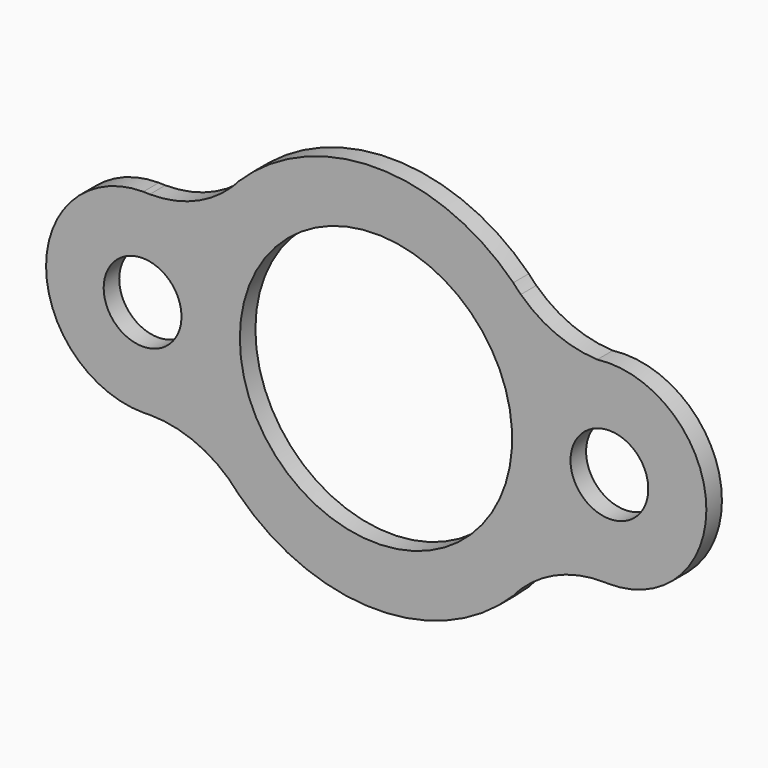
from build123d import *

# Parameters (mm, degrees)
F2_DEPTH = 6.35
F3_D     = 25.4
F4_D     = 88.9


# Not quite as in the source:
# - a length typed as a fraction of an inch, garbled in the dataset ("3 / 203.2 mm" for 3/8 in), is restored


with BuildPart() as f2:
    # F1 (on Front) → F2 (new body)
    with BuildSketch(Plane.XZ):
        with BuildLine():
            ThreePointArc((-47.2755417472, 42.3942574403), (-59.5317634989, 34.5003362533), (-73.8557984397, 31.7890660068))
            ThreePointArc((-73.8557984397, 31.7890660068), (-74.9040664455, 31.8092594153), (-75.9513814682, 31.8582984692))
            ThreePointArc((-75.9513814682, 31.8582984692), (-107.7013814682, 0.1082984692), (-75.9513814682, -31.6417015308))
            ThreePointArc((-75.9513814682, -31.6417015308), (-74.9868907208, -31.6001278987), (-74.0216562697, -31.5830041335))
            ThreePointArc((-74.0216562697, -31.5830041335), (-59.7325831056, -34.2859814401), (-47.4971337693, -42.1458464357))
            ThreePointArc((-47.4971337693, -42.1458464357), (-46.1209982776, -43.530970971), (-44.8176302016, -44.9847765041))
            ThreePointArc((-44.8176302016, -44.9847765041), (0, -63.5000010449), (44.8176302016, -44.9847765041))
            ThreePointArc((44.8176302016, -44.9847765041), (46.2263803756, -43.3976521369), (47.7215078569, -41.8916193935))
            ThreePointArc((47.7215078569, -41.8916193935), (60.0584421445, -34.0280617532), (74.4515791566, -31.4064032457))
            ThreePointArc((74.4515791566, -31.4064032457), (75.1167119815, -31.4211899869), (75.7814841371, -31.4476154228))
            ThreePointArc((75.7814841371, -31.4476154228), (107.7999571445, 2.0780448238), (72.2347193484, 31.814661464))
            ThreePointArc((72.2347193484, 31.814661464), (58.7820372427, 34.8087566031), (47.2755417472, 42.3942574403))
            ThreePointArc((47.2755417472, 42.3942574403), (46.0162162459, 43.6606882414), (44.8176431113, 44.9847615526))
            ThreePointArc((44.8176431113, 44.9847615526), (0, 63.4999989551), (-44.8176431113, 44.9847615526))
            ThreePointArc((-44.8176431113, 44.9847615526), (-46.0162162459, 43.6606882414), (-47.2755417472, 42.3942574403))
        make_face()
    extrude(amount=F2_DEPTH)

    # F3 (through all)
    with Locations(Plane(origin=(0, 0, 0), x_dir=(1, 0, 0), z_dir=(0, 1, 0))):
        with Locations((-76.2, 0), (76.2, 0)):
            Hole(F3_D / 2)

    # F4 (through all)
    with Locations(Plane(origin=(0, 0, 0), x_dir=(1, 0, 0), z_dir=(0, 1, 0))):
        with Locations((0, 0)):
            Hole(F4_D / 2)


solid = f2.part
